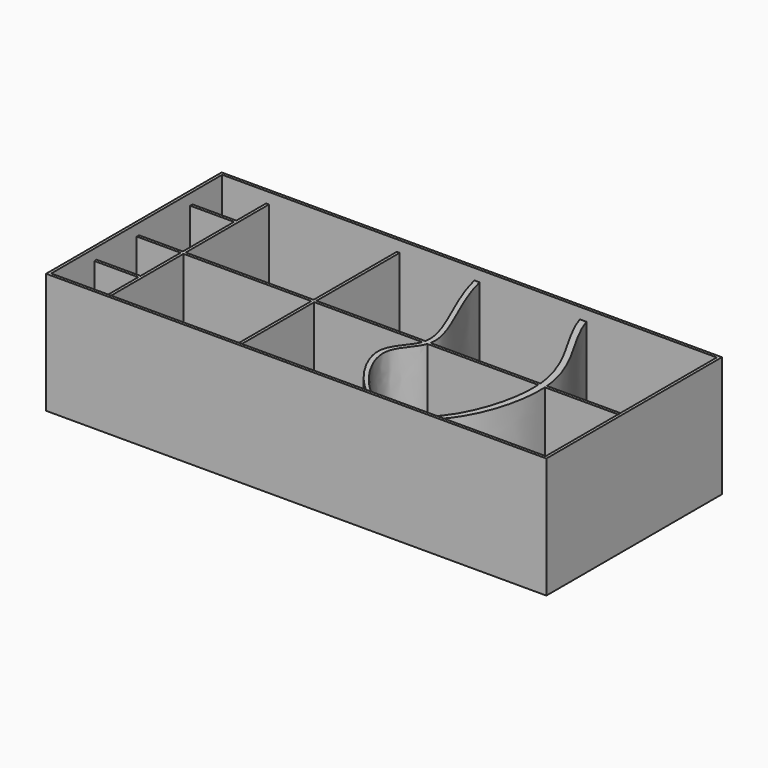
from build123d import *

# Parameters (mm, degrees)
F0_W     = 228
F0_H     = 100
F0_W_2   = 20
F0_H_2   = 24.5810076863
F0_H_3   = 22.8189926594
F0_H_4   = 29.1644897312
F0_W_3   = 58.2984770788
F0_H_5   = 47.4000003457
F0_H_6   = 16.9355106145
F1_DEPTH = 55
F2_W     = 225.4000006914
F2_H     = 97.4000006914
F3_DEPTH = 5


with BuildPart() as f1:
    # F0 (on Top) → F1 (new body)
    with BuildSketch(Plane.XY):
        with Locations((-66.3927308619, 15.6637772918)):
            Rectangle(F0_W, F0_H)
        with Locations((-169.0927312076, -20.7457192108)):
            Rectangle(F0_W_2, F0_H_2, mode=Mode.SUBTRACT)
        Polygon((-99.494241178, -33.0362230539), (-157.7927312076, -33.0362230539), (-157.7927312076, 15.6637772918), (-99.4942541288, 15.6637772918), align=None, mode=Mode.SUBTRACT)
        with Locations((-169.0927312076, 4.254280962)):
            Rectangle(F0_W_2, F0_H_3, mode=Mode.SUBTRACT)
        with BuildLine():
            add(Edge.make_bspline(
                [(-48.9903728661, 15.6637772918), (-50.8894876917, 10.2674604802), (-66.765290357, 1.4664925702), (-40.0663002403, -32.5316685311), (-25.9607383293, -33.0362230539)],
                knots=[0.2243177363, 0.2243177363, 0.2243177363, 0.2243177363, 0.3467822733, 0.5479791111, 0.5479791111, 0.5479791111, 0.5479791111], degree=3))
            Line((-25.9607383293, -33.0362230539), (-98.194241178, -33.0362230539))
            Line((-98.194241178, -33.0362230539), (-98.1942541288, 15.6637772918))
            Line((-98.1942541288, 15.6637772918), (-48.9903728661, 15.6637772918))
        make_face(mode=Mode.SUBTRACT)
        with BuildLine():
            add(Edge.make_bspline(
                [(-21.6105978481, -32.9644661853), (-6.3706766603, -31.3032384951), (5.0973679535, -4.3926706889), (3.8858228363, 15.6637772918)],
                knots=[0.5576009666, 0.5576009666, 0.5576009666, 0.5576009666, 0.7792958229, 0.7792958229, 0.7792958229, 0.7792958229], degree=3))
            add(Edge.make_bspline(
                [(-22.597104311, -33.0362230539), (-22.2665896559, -33.0241494524), (-21.9377248021, -33.0001246607), (-21.6105978481, -32.9644661853)],
                knots=[0.5528422567, 0.5528422567, 0.5528422567, 0.5528422567, 0.5576009666, 0.5576009666, 0.5576009666, 0.5576009666], degree=3))
            add(Edge.make_bspline(
                [(-23.6153104586, -33.0362230539), (-23.2743637388, -33.0484186836), (-22.9348725199, -33.0485616256), (-22.597104311, -33.0362230539)],
                knots=[0.5479791111, 0.5479791111, 0.5479791111, 0.5479791111, 0.5528422567, 0.5528422567, 0.5528422567, 0.5528422567], degree=3))
            add(Edge.make_bspline(
                [(-24.2891701926, -32.9966958469), (-24.0639725183, -33.0149937125), (-23.839327314, -33.0282099937), (-23.6153104586, -33.0362230539)],
                knots=[0.5447838124, 0.5447838124, 0.5447838124, 0.5447838124, 0.5479791111, 0.5479791111, 0.5479791111, 0.5479791111], degree=3))
            add(Edge.make_bspline(
                [(-46.6449449953, 15.6637772918), (-48.5440598209, 10.2674604802), (-64.2631309923, 1.5533788133), (-38.243886485, -31.8628407834), (-24.2891701926, -32.9966958469)],
                knots=[0.2243177363, 0.2243177363, 0.2243177363, 0.2243177363, 0.3467822733, 0.5447838124, 0.5447838124, 0.5447838124, 0.5447838124], degree=3))
            add(Edge.make_bspline(
                [(-46.2810248137, 16.9637772918), (-46.3742506197, 16.5161489966), (-46.4971600312, 16.0837068693), (-46.6449449953, 15.6637772918)],
                knots=[0.2147878138, 0.2147878138, 0.2147878138, 0.2147878138, 0.2243177363, 0.2243177363, 0.2243177363, 0.2243177363], degree=3))
            add(Edge.make_bspline(
                [(-61.7832280695, 64.3637776375), (-57.1571978586, 44.8554591392), (-44.1798779302, 27.0525374476), (-46.2810248137, 16.9637772918)],
                knots=[0, 0, 0, 0, 0.2147878138, 0.2147878138, 0.2147878138, 0.2147878138], degree=3))
            Line((-61.7832280695, 64.3637776375), (-58.7569419295, 64.3637776375))
            Line((-58.7569419295, 64.3637776375), (-18.4832829982, 64.3637776375))
            Line((-18.4832829982, 64.3637776375), (-16.1378551275, 64.3637776375))
            add(Edge.make_bspline(
                [(3.7889127405, 16.9637772918), (2.0816215591, 36.2077970929), (-11.2032608143, 49.1446081038), (-16.1378551275, 64.3637776375)],
                knots=[0.7841212321, 0.7841212321, 0.7841212321, 0.7841212321, 1, 1, 1, 1], degree=3))
            add(Edge.make_bspline(
                [(3.8858228363, 15.6637772918), (3.8594523508, 16.1003258471), (3.8270748012, 16.5336272046), (3.7889127405, 16.9637772918)],
                knots=[0.7792958229, 0.7792958229, 0.7792958229, 0.7792958229, 0.7841212321, 0.7841212321, 0.7841212321, 0.7841212321], degree=3))
        make_face(mode=Mode.SUBTRACT)
        with BuildLine():
            add(Edge.make_bspline(
                [(-19.5708181709, -33.0362230539), (-3.8425589006, -32.4616744452), (8.1496600722, -4.8231850372), (6.9121089764, 15.6637772918)],
                knots=[0.5528422567, 0.5528422567, 0.5528422567, 0.5528422567, 0.7792958229, 0.7792958229, 0.7792958229, 0.7792958229], degree=3))
            Line((6.9121089764, 15.6637772918), (46.3072694838, 15.6637772918))
            Line((46.3072694838, 15.6637772918), (46.3072694838, -33.0362230539))
            Line((46.3072694838, -33.0362230539), (-19.5708181709, -33.0362230539))
        make_face(mode=Mode.SUBTRACT)
        with Locations((-169.0927312076, 31.5460221574)):
            Rectangle(F0_W_2, F0_H_4, mode=Mode.SUBTRACT)
        with Locations((-128.6434926682, 40.6637774646)):
            Rectangle(F0_W_3, F0_H_5, mode=Mode.SUBTRACT)
        with Locations((-169.0927312076, 55.8960223302)):
            Rectangle(F0_W_2, F0_H_6, mode=Mode.SUBTRACT)
        with BuildLine():
            add(Edge.make_bspline(
                [(-64.1286559403, 64.3637776375), (-59.5026257294, 44.8554591392), (-46.525305801, 27.0525374476), (-48.6264526844, 16.9637772918)],
                knots=[0, 0, 0, 0, 0.2147878138, 0.2147878138, 0.2147878138, 0.2147878138], degree=3))
            Line((-48.6264526844, 16.9637772918), (-98.1942541288, 16.9637772918))
            Line((-98.1942541288, 16.9637772918), (-98.1942541288, 64.3637776375))
            Line((-98.1942541288, 64.3637776375), (-64.1286559403, 64.3637776375))
        make_face(mode=Mode.SUBTRACT)
        with BuildLine():
            Line((-13.1115689874, 64.3637776375), (46.3072694838, 64.3637776375))
            Line((46.3072694838, 64.3637776375), (46.3072694838, 16.9637772918))
            Line((46.3072694838, 16.9637772918), (6.8151988806, 16.9637772918))
            add(Edge.make_bspline(
                [(6.8151988806, 16.9637772918), (5.1079076992, 36.2077970929), (-8.1769746743, 49.1446081038), (-13.1115689874, 64.3637776375)],
                knots=[0.7841212321, 0.7841212321, 0.7841212321, 0.7841212321, 1, 1, 1, 1], degree=3))
        make_face(mode=Mode.SUBTRACT)
        with BuildLine():
            Line((1.5403949656, 15.6637772918), (3.8858228363, 15.6637772918))
            add(Edge.make_bspline(
                [(3.8858228363, 15.6637772918), (3.8594523508, 16.1003258471), (3.8270748012, 16.5336272046), (3.7889127405, 16.9637772918)],
                knots=[0.7792958229, 0.7792958229, 0.7792958229, 0.7792958229, 0.7841212321, 0.7841212321, 0.7841212321, 0.7841212321], degree=3))
            Line((3.7889127405, 16.9637772918), (1.4434848698, 16.9637772918))
            add(Edge.make_bspline(
                [(1.5403949656, 15.6637772918), (1.5140244801, 16.1003258471), (1.4816469304, 16.5336272046), (1.4434848698, 16.9637772918)],
                knots=[0.7792958229, 0.7792958229, 0.7792958229, 0.7792958229, 0.7841212321, 0.7841212321, 0.7841212321, 0.7841212321], degree=3))
        make_face()
        with BuildLine():
            Line((-43.6186588553, 15.6637772918), (1.5403949656, 15.6637772918))
            add(Edge.make_bspline(
                [(1.5403949656, 15.6637772918), (1.5140244801, 16.1003258471), (1.4816469304, 16.5336272046), (1.4434848698, 16.9637772918)],
                knots=[0.7792958229, 0.7792958229, 0.7792958229, 0.7792958229, 0.7841212321, 0.7841212321, 0.7841212321, 0.7841212321], degree=3))
            Line((1.4434848698, 16.9637772918), (-43.2547386736, 16.9637772918))
            add(Edge.make_bspline(
                [(-43.2547386736, 16.9637772918), (-43.3479644796, 16.5161489966), (-43.4708738911, 16.0837068693), (-43.6186588553, 15.6637772918)],
                knots=[0.2147878138, 0.2147878138, 0.2147878138, 0.2147878138, 0.2243177363, 0.2243177363, 0.2243177363, 0.2243177363], degree=3))
        make_face()
        with BuildLine():
            Line((-46.6449449953, 15.6637772918), (-43.6186588553, 15.6637772918))
            add(Edge.make_bspline(
                [(-43.2547386736, 16.9637772918), (-43.3479644796, 16.5161489966), (-43.4708738911, 16.0837068693), (-43.6186588553, 15.6637772918)],
                knots=[0.2147878138, 0.2147878138, 0.2147878138, 0.2147878138, 0.2243177363, 0.2243177363, 0.2243177363, 0.2243177363], degree=3))
            Line((-43.2547386736, 16.9637772918), (-46.2810248137, 16.9637772918))
            add(Edge.make_bspline(
                [(-46.2810248137, 16.9637772918), (-46.3742506197, 16.5161489966), (-46.4971600312, 16.0837068693), (-46.6449449953, 15.6637772918)],
                knots=[0.2147878138, 0.2147878138, 0.2147878138, 0.2147878138, 0.2243177363, 0.2243177363, 0.2243177363, 0.2243177363], degree=3))
        make_face()
    extrude(amount=F1_DEPTH)

    # F2 (on face) → F3 (cut)
    with BuildSketch(Plane.XY.offset(55)):
        with Locations((-66.3927308619, 15.6637772918)):
            Rectangle(F2_W, F2_H)
    extrude(amount=-F3_DEPTH, mode=Mode.SUBTRACT)


solid = f1.part
